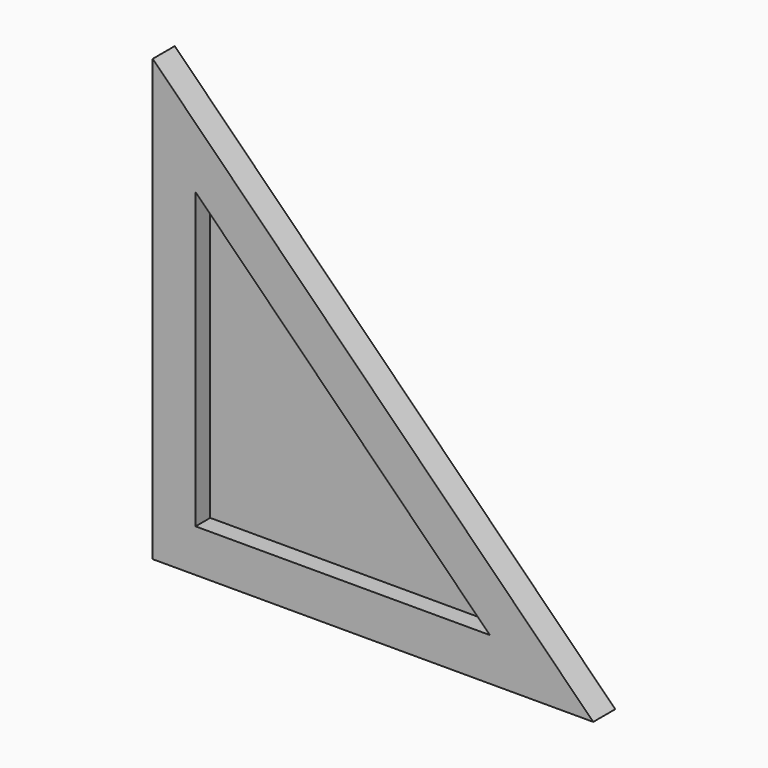
from build123d import *

# Parameters (mm, degrees)
F0_R     = 9.525
F1_DEPTH = 38.1
F2_DEPTH = 19.05


with BuildPart() as f1:
    # F0 (on Front) → F1 (new body)
    with BuildSketch(Plane.XZ):
        Polygon((914.4, 0), (0, 914.4), (0, 0), align=None)
        with Locations((44.45, 44.45)):
            Circle(F0_R, mode=Mode.SUBTRACT)
        Polygon((699.776414305, 88.9), (88.9, 88.9), (88.9, 699.776414305), align=None, mode=Mode.SUBTRACT)
        with Locations((44.45, 44.45)):
            Circle(F0_R)
    extrude(amount=F1_DEPTH)

    # F0 (on Front) → F2 (join)
    with BuildSketch(Plane.XZ):
        Polygon((914.4, 0), (0, 914.4), (0, 0), align=None)
        with Locations((44.45, 44.45)):
            Circle(F0_R, mode=Mode.SUBTRACT)
        Polygon((699.776414305, 88.9), (88.9, 88.9), (88.9, 699.776414305), align=None, mode=Mode.SUBTRACT)
        Polygon((88.9, 699.776414305), (88.9, 88.9), (699.776414305, 88.9), align=None)
        with Locations((44.45, 44.45)):
            Circle(F0_R)
    extrude(amount=-F2_DEPTH)


solid = f1.part
